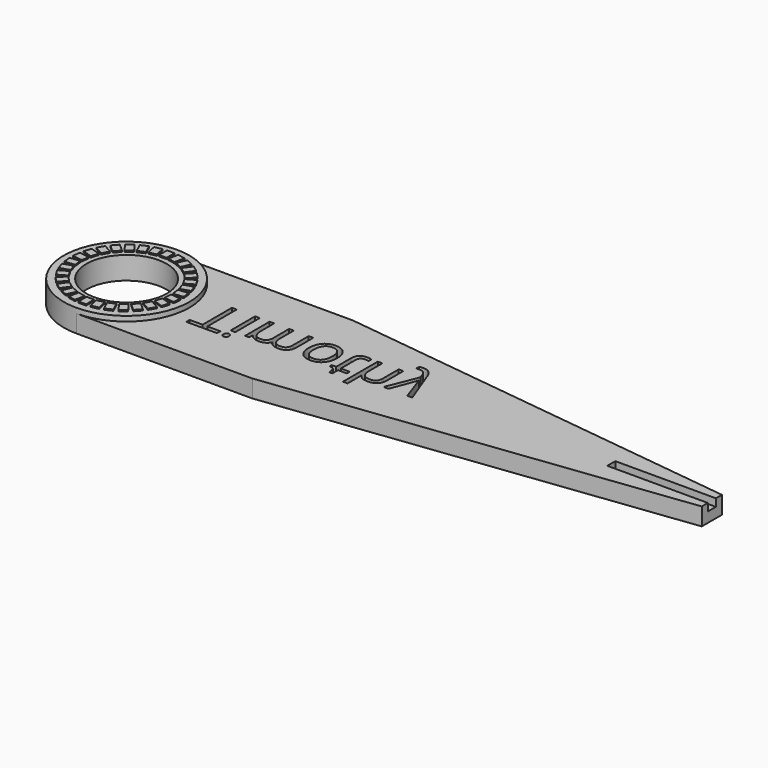
from build123d import *

# Parameters (mm, degrees)
F0_R         = 8
F1_DEPTH     = 3.5
F2_R         = 12.5
F2_R_2       = 8
F3_DEPTH     = 1
F4_W         = 1.5
F4_H         = 2
F5_DEPTH     = 0.25
F6_W         = 20
F6_H         = 2
F7_DEPTH     = 1.5
F9_TEXT_SIZE = 11.394436003
F10_DEPTH    = 3.501


# Not quite as in the source:
# - Text() gives the source's letters only with a copy of the font that has no kerning and outlines rounded to 1/6400 em; it was checked with that copy


with BuildPart() as f1:
    # F0 (on Top) → F1 (new body)
    with BuildSketch(Plane.XY):
        with BuildLine():
            Line((35, 12.5), (0, 12.5))
            ThreePointArc((0, 12.5), (-12.5, 0), (0, -12.5))
            Line((0, -12.5), (35, -12.5))
            Line((35, -12.5), (116.3887844346, -2.5067138408))
            Line((116.3887844346, -2.5067138408), (116.3887844346, 2.5067138408))
            Line((116.3887844346, 2.5067138408), (35, 12.5))
        make_face()
        Circle(F0_R, mode=Mode.SUBTRACT)
    extrude(amount=F1_DEPTH)

    # F2 (on face) → F3 (join)
    with BuildSketch(Plane.XY.offset(3.5)):
        Circle(F2_R)
        Circle(F2_R_2, mode=Mode.SUBTRACT)
    extrude(amount=F3_DEPTH)

    # F4 (on face) → F5 (join)
    with BuildSketch(Plane.XY.offset(4.5)):
        with Locations((0, 10)):
            Rectangle(F4_W, F4_H)
        Polygon((-3.0206392995, 10.60368984), (-2.6048159179, 8.6473946385), (-1.1375945168, 8.9592621747), (-1.5534178984, 10.9155573762), align=None)
        Polygon((-5.1592621671, 9.7439475518), (-4.3457888809, 7.9168566365), (-2.9754706945, 8.5269616011), (-3.7889439806, 10.3540525164), align=None)
        Polygon((-7.072400521, 8.4583479989), (-5.8968300164, 6.8403140102), (-4.6833045249, 7.7219918886), (-5.8588750294, 9.3400258773), align=None)
        Polygon((-8.676441035, 6.8030780508), (-7.1901513841, 5.4648168381), (-6.1864554745, 6.5795340763), (-7.6727451255, 7.9177952891), align=None)
        Polygon((-9.9012794416, 4.8504809472), (-8.1692286341, 3.8504809472), (-7.4192286341, 5.1495190528), (-9.1512794416, 6.1495190528), align=None)
        Polygon((-10.693384425, 2.6858945509), (-8.7912713924, 2.0678605622), (-8.3277459009, 3.4944453366), (-10.2298589335, 4.1124793253), align=None)
        Polygon((-11.0181371965, 0.4039216744), (-9.0290934058, 0.1948647479), (-8.8723007109, 1.6866475909), (-10.8613445016, 1.8957045175), align=None)
        Polygon((-10.8613445016, -1.8957045175), (-8.8723007109, -1.6866475909), (-9.0290934058, -0.1948647479), (-11.0181371965, -0.4039216744), align=None)
        Polygon((-10.2298589335, -4.1124793253), (-8.3277459009, -3.4944453366), (-8.7912713924, -2.0678605622), (-10.693384425, -2.6858945509), align=None)
        Polygon((-9.1512794416, -6.1495190528), (-7.4192286341, -5.1495190528), (-8.1692286341, -3.8504809472), (-9.9012794416, -4.8504809472), align=None)
        Polygon((-7.6727451255, -7.9177952891), (-6.1864554745, -6.5795340763), (-7.1901513841, -5.4648168381), (-8.676441035, -6.8030780508), align=None)
        Polygon((-5.8588750294, -9.3400258773), (-4.6833045249, -7.7219918886), (-5.8968300164, -6.8403140102), (-7.072400521, -8.4583479989), align=None)
        Polygon((-3.7889439806, -10.3540525164), (-2.9754706945, -8.5269616011), (-4.3457888809, -7.9168566365), (-5.1592621671, -9.7439475518), align=None)
        Polygon((-1.5534178984, -10.9155573762), (-1.1375945168, -8.9592621747), (-2.6048159179, -8.6473946385), (-3.0206392995, -10.60368984), align=None)
        with Locations((0, -10)):
            Rectangle(F4_W, F4_H)
        Polygon((3.0206392995, -10.60368984), (2.6048159179, -8.6473946385), (1.1375945168, -8.9592621747), (1.5534178984, -10.9155573762), align=None)
        Polygon((5.1592621671, -9.7439475518), (4.3457888809, -7.9168566365), (2.9754706945, -8.5269616011), (3.7889439806, -10.3540525164), align=None)
        Polygon((7.072400521, -8.4583479989), (5.8968300164, -6.8403140102), (4.6833045249, -7.7219918886), (5.8588750294, -9.3400258773), align=None)
        Polygon((8.676441035, -6.8030780508), (7.1901513841, -5.4648168381), (6.1864554745, -6.5795340763), (7.6727451255, -7.9177952891), align=None)
        Polygon((9.9012794416, -4.8504809472), (8.1692286341, -3.8504809472), (7.4192286341, -5.1495190528), (9.1512794416, -6.1495190528), align=None)
        Polygon((10.693384425, -2.6858945509), (8.7912713924, -2.0678605622), (8.3277459009, -3.4944453366), (10.2298589335, -4.1124793253), align=None)
        Polygon((11.0181371965, -0.4039216744), (9.0290934058, -0.1948647479), (8.8723007109, -1.6866475909), (10.8613445016, -1.8957045175), align=None)
        Polygon((10.8613445016, 1.8957045175), (8.8723007109, 1.6866475909), (9.0290934058, 0.1948647479), (11.0181371965, 0.4039216744), align=None)
        Polygon((10.2298589335, 4.1124793253), (8.3277459009, 3.4944453366), (8.7912713924, 2.0678605622), (10.693384425, 2.6858945509), align=None)
        Polygon((9.1512794416, 6.1495190528), (7.4192286341, 5.1495190528), (8.1692286341, 3.8504809472), (9.9012794416, 4.8504809472), align=None)
        Polygon((7.6727451255, 7.9177952891), (6.1864554745, 6.5795340763), (7.1901513841, 5.4648168381), (8.676441035, 6.8030780508), align=None)
        Polygon((5.8588750294, 9.3400258773), (4.6833045249, 7.7219918886), (5.8968300164, 6.8403140102), (7.072400521, 8.4583479989), align=None)
        Polygon((3.7889439806, 10.3540525164), (2.9754706945, 8.5269616011), (4.3457888809, 7.9168566365), (5.1592621671, 9.7439475518), align=None)
        Polygon((1.5534178984, 10.9155573762), (1.1375945168, 8.9592621747), (2.6048159179, 8.6473946385), (3.0206392995, 10.60368984), align=None)
    extrude(amount=F5_DEPTH)

    # F6 (on face) → F7 (cut)
    with BuildSketch(Plane.XY.offset(3.5)):
        with Locations((106.3887844346, 0.0067138408)):
            Rectangle(F6_W, F6_H)
    extrude(amount=-F7_DEPTH, mode=Mode.SUBTRACT)

    # F9 (on face) → F10 (cut, through all)
    with BuildSketch(Plane(origin=(0, 0, 3.5), x_dir=(1, 0, 0), z_dir=(0, 0, -1))):
        with Locations((15, -4.1019969611)):
            Text('Timothy', F9_TEXT_SIZE, font='Open Sans', text_align=(TextAlign.LEFT, TextAlign.BOTTOM))
    extrude(amount=F10_DEPTH, mode=Mode.SUBTRACT)


solid = f1.part
